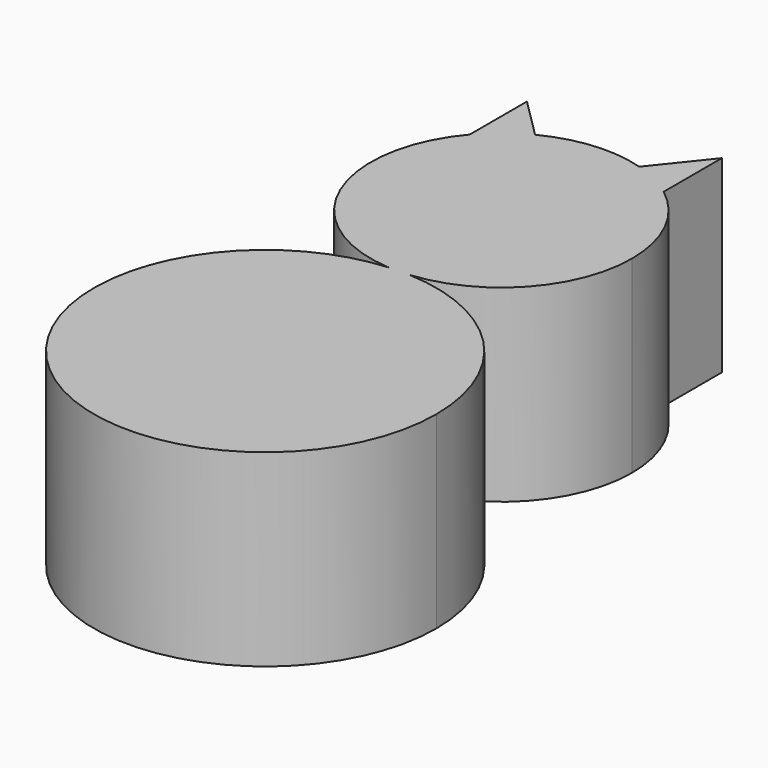
from build123d import *

# Parameters (mm, degrees)
F0_R     = 3.3666282328
F0_R_2   = 4.2780726565
F1_DEPTH = 25.4


with BuildPart() as f1:
    # F0 (on Top) → F1 (new body)
    with BuildSketch(Plane.XY):
        with BuildLine():
            ThreePointArc((-22.1343814945, 32.3195395849), (-10.7773284043, 37.9899650978), (-6.1959977362, 49.8283682714))
            ThreePointArc((-6.1959977362, 49.8283682714), (-8.017979687, 57.6234855899), (-13.1064001471, 63.8034086848))
            ThreePointArc((-13.1064001471, 63.8034086848), (-15.7610771081, 65.4788003499), (-18.6713267733, 66.6555305166))
            ThreePointArc((-18.6713267733, 66.6555305166), (-25.3338728535, 67.3459786854), (-31.771318173, 65.4951581371))
            ThreePointArc((-31.771318173, 65.4951581371), (-34.6785879171, 63.6321004456), (-37.1657780069, 61.236878789))
            ThreePointArc((-37.1657780069, 61.236878789), (-39.9749449815, 42.9676641594), (-24.8959708176, 32.2774742434))
            ThreePointArc((-24.8959708176, 32.2774742434), (-23.515806874, 32.3399135434), (-22.1343814945, 32.3195395849))
        make_face()
        with Locations((-33.5280001163, 56.845203042)):
            Circle(F0_R, mode=Mode.SUBTRACT)
        with Locations((-18.897600472, 56.845203042)):
            Circle(F0_R_2, mode=Mode.SUBTRACT)
        with BuildLine():
            ThreePointArc((-18.6713267733, 66.6555305166), (-15.7610771081, 65.4788003499), (-13.1064001471, 63.8034086848))
            Line((-13.1064001471, 63.8034086848), (-13.1064001471, 73.6092031002))
            Line((-13.1064001471, 73.6092031002), (-18.6713267733, 66.6555305166))
        make_face()
        with BuildLine():
            ThreePointArc((-3.572438767, 21.4317220567), (-11.5045727225, 29.1751773236), (-22.1343814945, 32.3195395849))
            ThreePointArc((-22.1343814945, 32.3195395849), (-23.5143490847, 32.2442096875), (-24.8959708176, 32.2774742434))
            ThreePointArc((-24.8959708176, 32.2774742434), (-35.1264416512, 28.9952801275), (-42.7571638322, 21.4317220567))
            ThreePointArc((-42.7571638322, 21.4317220567), (-29.4734249224, -12.8695185824), (-0.1186150736, 9.2964004725))
            ThreePointArc((-0.1186150736, 9.2964004725), (-0.9988822447, 15.6050240953), (-3.572438767, 21.4317220567))
        make_face()
        with BuildLine():
            ThreePointArc((-24.8959708176, 32.2774742434), (-23.5143490847, 32.2442096875), (-22.1343814945, 32.3195395849))
            ThreePointArc((-22.1343814945, 32.3195395849), (-23.515806874, 32.3399135434), (-24.8959708176, 32.2774742434))
        make_face()
        with BuildLine():
            ThreePointArc((-37.1657780069, 61.236878789), (-34.6785879171, 63.6321004456), (-31.771318173, 65.4951581371))
            Line((-31.771318173, 65.4951581371), (-37.1657780069, 70.8660041886))
            Line((-37.1657780069, 70.8660041886), (-37.1657780069, 61.236878789))
        make_face()
        with Locations((-33.5280001163, 56.845203042)):
            Circle(F0_R)
        with Locations((-18.897600472, 56.845203042)):
            Circle(F0_R_2)
    extrude(amount=F1_DEPTH)


solid = f1.part
